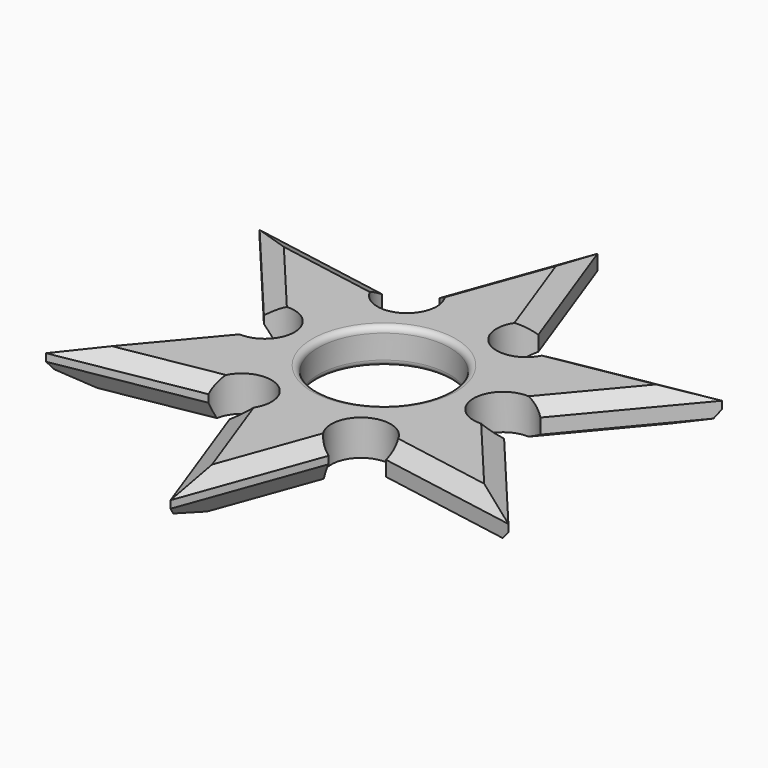
from build123d import *

# Parameters (mm, degrees)
F0_R         = 11.1
F1_DEPTH     = 6
F2_C1_SIZE2  = 3
F2_C1_SIZE   = 1.7320508076
F2_C2_SIZE2  = 3
F2_C2_SIZE   = 1.7320508076
F2_C3_SIZE2  = 3
F2_C3_SIZE   = 1.7320508076
F2_C4_SIZE2  = 3
F2_C4_SIZE   = 1.7320508076
F2_C5_SIZE2  = 1.7320508076
F2_C5_SIZE   = 3
F2_C6_SIZE2  = 3
F2_C6_SIZE   = 1.7320508076
F2_C7_SIZE2  = 1.7320508076
F2_C7_SIZE   = 3
F2_C8_SIZE2  = 3
F2_C8_SIZE   = 1.7320508076
F2_C9_SIZE2  = 1.7320508076
F2_C9_SIZE   = 3
F2_C10_SIZE2 = 3
F2_C10_SIZE  = 1.7320508076
F2_C11_SIZE2 = 3
F2_C11_SIZE  = 1.7320508076
F2_C12_SIZE2 = 3
F2_C12_SIZE  = 1.7320508076
F2_C13_SIZE2 = 1.7320508076
F2_C13_SIZE  = 3
F2_C14_SIZE2 = 3
F2_C14_SIZE  = 1.7320508076
F2_C15_SIZE2 = 3
F2_C15_SIZE  = 1.7320508076
F2_C16_SIZE2 = 3
F2_C16_SIZE  = 1.7320508076
F2_C17_SIZE2 = 1.7320508076
F2_C17_SIZE  = 3
F2_C18_SIZE2 = 3
F2_C18_SIZE  = 1.7320508076
F2_C19_SIZE2 = 3
F2_C19_SIZE  = 1.7320508076
F2_C20_SIZE2 = 3
F2_C20_SIZE  = 1.7320508076
F2_C21_SIZE2 = 1.7320508076
F2_C21_SIZE  = 3
F2_C22_SIZE2 = 3
F2_C22_SIZE  = 1.7320508076
F2_C23_SIZE2 = 3
F2_C23_SIZE  = 1.7320508076
F2_C24_SIZE2 = 3
F2_C24_SIZE  = 1.7320508076
F3_R         = 1


with BuildPart() as f1:
    # F0 (on Top) → F1 (new body)
    with BuildSketch(Plane.XY):
        with BuildLine():
            Line((8.3388454559, 22.1051900243), (0, 45))
            Line((0, 45), (-8.3388454559, 22.1051900243))
            ThreePointArc((-8.3388454559, 22.1051900243), (-7.55, 13.0769835971), (-14.9742333886, 18.2742470152))
            Line((-14.9742333886, 18.2742470152), (-38.9711431703, 22.5))
            Line((-38.9711431703, 22.5), (-23.3130788445, 3.8309430091))
            ThreePointArc((-23.3130788445, 3.8309430091), (-15.1, 0), (-23.3130788445, -3.8309430091))
            Line((-23.3130788445, -3.8309430091), (-38.9711431703, -22.5))
            Line((-38.9711431703, -22.5), (-14.9742333886, -18.2742470152))
            ThreePointArc((-14.9742333886, -18.2742470152), (-7.55, -13.0769835971), (-8.3388454559, -22.1051900243))
            Line((-8.3388454559, -22.1051900243), (0, -45))
            Line((0, -45), (8.3388454559, -22.1051900243))
            ThreePointArc((8.3388454559, -22.1051900243), (7.55, -13.0769835971), (14.9742333886, -18.2742470152))
            Line((14.9742333886, -18.2742470152), (38.9711431703, -22.5))
            Line((38.9711431703, -22.5), (23.3130788445, -3.8309430091))
            ThreePointArc((23.3130788445, -3.8309430091), (15.1, 0), (23.3130788445, 3.8309430091))
            Line((23.3130788445, 3.8309430091), (38.9711431703, 22.5))
            Line((38.9711431703, 22.5), (14.9742333886, 18.2742470152))
            ThreePointArc((14.9742333886, 18.2742470152), (7.55, 13.0769835971), (8.3388454559, 22.1051900243))
        make_face()
        Circle(F0_R, mode=Mode.SUBTRACT)
    extrude(amount=F1_DEPTH)

    # F2: chamfer of 3 x 1.7320508076 on 24 edges, made by hand

    # F2_c1
    f2_c1_edges = [f1.edges().sort_by_distance(p)[0] for p in [
        (31.1421110074, 13.1654715045, 0),
    ]]
    f2_c1_side = f1.faces().sort_by_distance((31.1421110074, 13.1654715045, 0.0346410162))[0]
    chamfer(f2_c1_edges, length=F2_C1_SIZE, length2=F2_C1_SIZE2, reference=f2_c1_side)

    # F2_c2
    f2_c2_edges = [f1.edges().sort_by_distance(p)[0] for p in [
        (31.1421110074, 13.1654715045, 6),
    ]]
    f2_c2_side = f1.faces().sort_by_distance((31.1421110074, 13.1654715045, 5.9653589838))[0]
    chamfer(f2_c2_edges, length=F2_C2_SIZE, length2=F2_C2_SIZE2, reference=f2_c2_side)

    # F2_c3
    f2_c3_edges = [f1.edges().sort_by_distance(p)[0] for p in [
        (24.6756919125, 19.9826322901, 0),
    ]]
    f2_c3_side = f1.faces().sort_by_distance((24.6816996097, 19.9485162005, 0))[0]
    chamfer(f2_c3_edges, length=F2_C3_SIZE, length2=F2_C3_SIZE2, reference=f2_c3_side)

    # F2_c4
    f2_c4_edges = [f1.edges().sort_by_distance(p)[0] for p in [
        (24.6756919125, 19.9826322901, 6),
    ]]
    f2_c4_side = f1.faces().sort_by_distance((24.6756919125, 19.9826322901, 5.9653589838))[0]
    chamfer(f2_c4_edges, length=F2_C4_SIZE, length2=F2_C4_SIZE2, reference=f2_c4_side)

    # F2_c5
    f2_c5_edges = [f1.edges().sort_by_distance(p)[0] for p in [
        (4.169422728, 33.5525950122, 0),
    ]]
    f2_c5_side = f1.faces().sort_by_distance((4.136873479, 33.5407397857, 0))[0]
    chamfer(f2_c5_edges, length=F2_C5_SIZE, length2=F2_C5_SIZE2, reference=f2_c5_side)

    # F2_c6
    f2_c6_edges = [f1.edges().sort_by_distance(p)[0] for p in [
        (4.169422728, 33.5525950122, 6),
    ]]
    f2_c6_side = f1.faces().sort_by_distance((4.169422728, 33.5525950122, 5.9653589838))[0]
    chamfer(f2_c6_edges, length=F2_C6_SIZE, length2=F2_C6_SIZE2, reference=f2_c6_side)

    # F2_c7
    f2_c7_edges = [f1.edges().sort_by_distance(p)[0] for p in [
        (-4.9676212415, 31.3610921973, 0),
    ]]
    f2_c7_side = f1.faces().sort_by_distance((-4.9350719925, 31.3492369708, 0))[0]
    chamfer(f2_c7_edges, length=F2_C7_SIZE, length2=F2_C7_SIZE2, reference=f2_c7_side)

    # F2_c8
    f2_c8_edges = [f1.edges().sort_by_distance(p)[0] for p in [
        (-4.9676212415, 31.3610921973, 6),
    ]]
    f2_c8_side = f1.faces().sort_by_distance((-4.9676212415, 31.3610921973, 5.9653589838))[0]
    chamfer(f2_c8_edges, length=F2_C8_SIZE, length2=F2_C8_SIZE2, reference=f2_c8_side)

    # F2_c9
    f2_c9_edges = [f1.edges().sort_by_distance(p)[0] for p in [
        (-26.9726882794, 20.3871235076, 0),
    ]]
    f2_c9_side = f1.faces().sort_by_distance((-26.9786959766, 20.353007418, 0))[0]
    chamfer(f2_c9_edges, length=F2_C9_SIZE, length2=F2_C9_SIZE2, reference=f2_c9_side)

    # F2_c10
    f2_c10_edges = [f1.edges().sort_by_distance(p)[0] for p in [
        (-26.9726882794, 20.3871235076, 6),
    ]]
    f2_c10_side = f1.faces().sort_by_distance((-26.9726882794, 20.3871235076, 5.9653589838))[0]
    chamfer(f2_c10_edges, length=F2_C10_SIZE, length2=F2_C10_SIZE2, reference=f2_c10_side)

    # F2_c11
    f2_c11_edges = [f1.edges().sort_by_distance(p)[0] for p in [
        (-29.643313154, 11.3784599071, 0),
    ]]
    f2_c11_side = f1.faces().sort_by_distance((-29.6167716023, 11.4007207704, 0))[0]
    chamfer(f2_c11_edges, length=F2_C11_SIZE, length2=F2_C11_SIZE2, reference=f2_c11_side)

    # F2_c12
    f2_c12_edges = [f1.edges().sort_by_distance(p)[0] for p in [
        (-29.643313154, 11.3784599071, 6),
    ]]
    f2_c12_side = f1.faces().sort_by_distance((-29.643313154, 11.3784599071, 5.9653589838))[0]
    chamfer(f2_c12_edges, length=F2_C12_SIZE, length2=F2_C12_SIZE2, reference=f2_c12_side)

    # F2_c13
    f2_c13_edges = [f1.edges().sort_by_distance(p)[0] for p in [
        (-31.1421110074, -13.1654715045, 0),
    ]]
    f2_c13_side = f1.faces().sort_by_distance((-31.1155694557, -13.1877323678, 0))[0]
    chamfer(f2_c13_edges, length=F2_C13_SIZE, length2=F2_C13_SIZE2, reference=f2_c13_side)

    # F2_c14
    f2_c14_edges = [f1.edges().sort_by_distance(p)[0] for p in [
        (-31.1421110074, -13.1654715045, 6),
    ]]
    f2_c14_side = f1.faces().sort_by_distance((-31.1421110074, -13.1654715045, 5.9653589838))[0]
    chamfer(f2_c14_edges, length=F2_C14_SIZE, length2=F2_C14_SIZE2, reference=f2_c14_side)

    # F2_c15
    f2_c15_edges = [f1.edges().sort_by_distance(p)[0] for p in [
        (-24.6756919125, -19.9826322901, 0),
    ]]
    f2_c15_side = f1.faces().sort_by_distance((-24.6816996097, -19.9485162005, 0))[0]
    chamfer(f2_c15_edges, length=F2_C15_SIZE, length2=F2_C15_SIZE2, reference=f2_c15_side)

    # F2_c16
    f2_c16_edges = [f1.edges().sort_by_distance(p)[0] for p in [
        (-24.6756919125, -19.9826322901, 6),
    ]]
    f2_c16_side = f1.faces().sort_by_distance((-24.6756919125, -19.9826322901, 5.9653589838))[0]
    chamfer(f2_c16_edges, length=F2_C16_SIZE, length2=F2_C16_SIZE2, reference=f2_c16_side)

    # F2_c17
    f2_c17_edges = [f1.edges().sort_by_distance(p)[0] for p in [
        (-4.169422728, -33.5525950122, 0),
    ]]
    f2_c17_side = f1.faces().sort_by_distance((-4.136873479, -33.5407397857, 0))[0]
    chamfer(f2_c17_edges, length=F2_C17_SIZE, length2=F2_C17_SIZE2, reference=f2_c17_side)

    # F2_c18
    f2_c18_edges = [f1.edges().sort_by_distance(p)[0] for p in [
        (-4.169422728, -33.5525950122, 6),
    ]]
    f2_c18_side = f1.faces().sort_by_distance((-4.169422728, -33.5525950122, 5.9653589838))[0]
    chamfer(f2_c18_edges, length=F2_C18_SIZE, length2=F2_C18_SIZE2, reference=f2_c18_side)

    # F2_c19
    f2_c19_edges = [f1.edges().sort_by_distance(p)[0] for p in [
        (4.9676212415, -31.3610921973, 0),
    ]]
    f2_c19_side = f1.faces().sort_by_distance((4.9350719925, -31.3492369708, 0))[0]
    chamfer(f2_c19_edges, length=F2_C19_SIZE, length2=F2_C19_SIZE2, reference=f2_c19_side)

    # F2_c20
    f2_c20_edges = [f1.edges().sort_by_distance(p)[0] for p in [
        (4.9676212415, -31.3610921973, 6),
    ]]
    f2_c20_side = f1.faces().sort_by_distance((4.9676212415, -31.3610921973, 5.9653589838))[0]
    chamfer(f2_c20_edges, length=F2_C20_SIZE, length2=F2_C20_SIZE2, reference=f2_c20_side)

    # F2_c21
    f2_c21_edges = [f1.edges().sort_by_distance(p)[0] for p in [
        (26.9726882794, -20.3871235076, 0),
    ]]
    f2_c21_side = f1.faces().sort_by_distance((26.9786959766, -20.353007418, 0))[0]
    chamfer(f2_c21_edges, length=F2_C21_SIZE, length2=F2_C21_SIZE2, reference=f2_c21_side)

    # F2_c22
    f2_c22_edges = [f1.edges().sort_by_distance(p)[0] for p in [
        (26.9726882794, -20.3871235076, 6),
    ]]
    f2_c22_side = f1.faces().sort_by_distance((26.9726882794, -20.3871235076, 5.9653589838))[0]
    chamfer(f2_c22_edges, length=F2_C22_SIZE, length2=F2_C22_SIZE2, reference=f2_c22_side)

    # F2_c23
    f2_c23_edges = [f1.edges().sort_by_distance(p)[0] for p in [
        (29.643313154, -11.3784599071, 0),
    ]]
    f2_c23_side = f1.faces().sort_by_distance((29.6167716023, -11.4007207704, 0))[0]
    chamfer(f2_c23_edges, length=F2_C23_SIZE, length2=F2_C23_SIZE2, reference=f2_c23_side)

    # F2_c24
    f2_c24_edges = [f1.edges().sort_by_distance(p)[0] for p in [
        (29.643313154, -11.3784599071, 6),
    ]]
    f2_c24_side = f1.faces().sort_by_distance((29.643313154, -11.3784599071, 5.9653589838))[0]
    chamfer(f2_c24_edges, length=F2_C24_SIZE, length2=F2_C24_SIZE2, reference=f2_c24_side)

    # F3
    f3_edges = [f1.edges().sort_by_distance(p)[0] for p in [
        (-11.1, 0, 0),
        (-11.1, 0, 6),
    ]]
    fillet(f3_edges, radius=F3_R)


solid = f1.part
